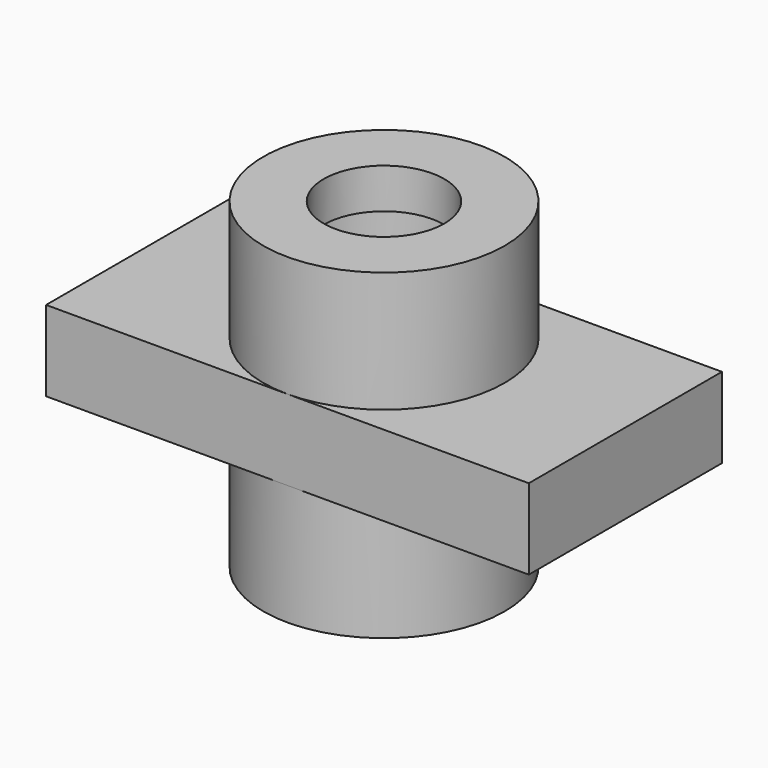
from build123d import *

# Parameters (mm, degrees)
F3_W = 38.1
F3_H = 12.7


# Not quite as in the source:
# - a pattern or mirror of a feature is missing from the dataset's text; its kind, count and spacing are read off the source's solid


with BuildPart() as f1:
    # F0 (on Front) → F1 (revolve)
    with BuildSketch(Plane.XZ):
        Polygon((9.525, 38.1), (9.525, 0), (19.05, 0), (19.05, 50.8), (9.525, 50.8), (9.525, 44.45), (12.7, 44.45), (12.7, 38.1), align=None)
    revolve(axis=Axis((0, 0, 18.9327914268), (0, 0, 1)))

    # F3 (on offset) → F4 (join, up to the next surface of F1)
    with BuildSketch(Plane.YZ.offset(38.1)):
        with Locations((0, 25.4)):
            Rectangle(F3_W, F3_H)
    f4 = extrude(until=Until.NEXT, dir=(-1, 0, 0))

    # F4_copies: F4 across plane
    add(f4.mirror(Plane(origin=(0, 0, 0), x_dir=(0, 0, -1), z_dir=(-1, 0, 0))))


solid = f1.part
